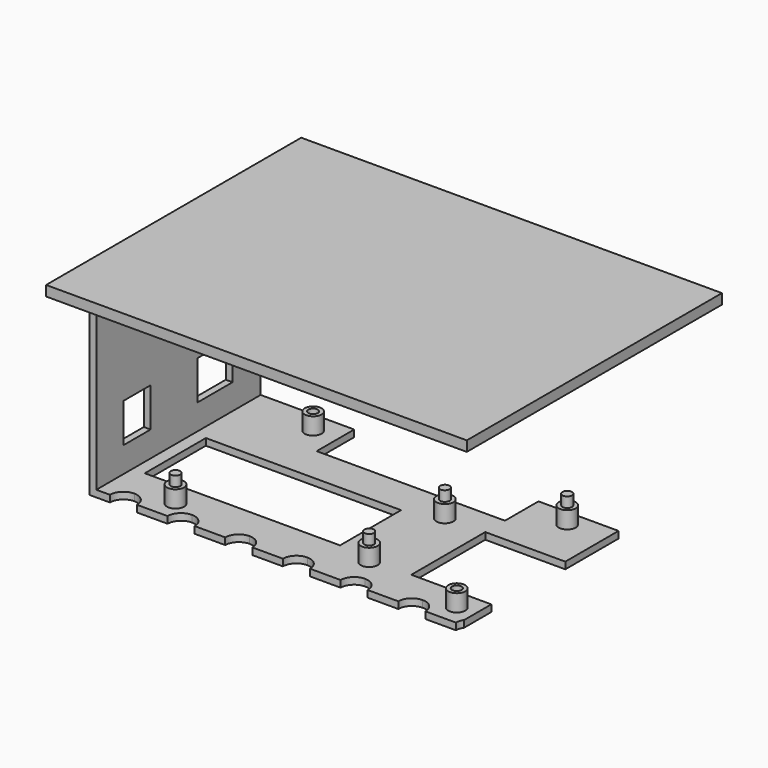
from build123d import *

# Parameters (mm, degrees)
F0_W      = 124
F0_H      = 94
F1_DEPTH  = 2
F2_DEPTH  = 58
F3_R      = 2.5
F4_DEPTH  = 5
F5_R      = 1.4
F6_DEPTH  = 3
F7_D      = 2.8
F7_DEPTH  = 5
F7_TIP    = 0.8412048666
F9_DEPTH  = 8
F10_W     = 1
F10_H     = 50
F11_DEPTH = 3
F12_W     = 5
F12_H     = 3
F13_DEPTH = 1
F14_W     = 124
F14_H     = 94
F15_DEPTH = 3
F17_W     = 2
F17_H     = 13
F17_H_2   = 10
F18_DEPTH = 11.5
F19_W     = 199.5194256306
F19_H     = 143.535412848
F19_W_2   = 57.5444861315
F19_H_2   = 22.4794349963
F20_DEPTH = 100


# Not quite as in the source:
# - a feature names something its author has since deleted; it is built from what else it names


with BuildPart() as f1:
    # F0 (on Top) → F1 (new body)
    with BuildSketch(Plane.XY):
        Rectangle(F0_W, F0_H)
        Polygon((-60, -45), (-60, 45), (60, 45), (60, 31), (60, 29), (60, -45), align=None, mode=Mode.SUBTRACT)
        Polygon((60, 45), (-60, 45), (-60, -45), (60, -45), (60, 29), (60, 31), align=None)
    extrude(amount=F1_DEPTH)

    # F0 (on Top) → F2 (join)
    with BuildSketch(Plane.XY):
        Rectangle(F0_W, F0_H)
        Polygon((-60, -45), (-60, 45), (60, 45), (60, 31), (60, 29), (60, -45), align=None, mode=Mode.SUBTRACT)
    extrude(amount=F2_DEPTH)

    # F3 (on face) → F4 (join)
    with BuildSketch(Plane.XY.offset(2)):
        with Locations((35.45, 23.2)):
            Circle(F3_R)
        with Locations((11.55, -19.9)):
            Circle(F3_R)
        with Locations((41.45, -25)):
            Circle(F3_R)
        with Locations((11.55, 8)):
            Circle(F3_R)
        with Locations((-39.45, 23.2)):
            Circle(F3_R)
        with Locations((-41.45, -25)):
            Circle(F3_R)
    extrude(amount=F4_DEPTH)

    # F5 (on face) → F6 (join)
    with BuildSketch(Plane.XY.offset(7)):
        with Locations((35.45, 23.2)):
            Circle(F5_R)
        with Locations((11.55, 8)):
            Circle(F5_R)
        with Locations((11.55, -19.9)):
            Circle(F5_R)
        with Locations((-41.45, -25)):
            Circle(F5_R)
    extrude(amount=F6_DEPTH)

    # F7 (one way)
    with BuildSketch(Plane(origin=(0, 0, 2), x_dir=(1, 0, 0), z_dir=(0, 0, -1))):
        with Locations((-39.45, -23.2), (41.45, 25)):
            Circle(F7_D / 2)
    extrude(amount=-F7_DEPTH, mode=Mode.SUBTRACT)
    with Locations(Plane(origin=(0, 0, 2), x_dir=(1, 0, 0), z_dir=(0, 0, -1))):
        with Locations((-39.45, -23.2), (41.45, 25)):
            with Locations((0, 0, -(F7_DEPTH + F7_TIP / 2))):  # 118° drill point
                Cone(0, F7_D / 2, F7_TIP, mode=Mode.SUBTRACT)

    # F8 (on face) → F9 (cut)
    with BuildSketch(Plane(origin=(0, 0, 0), x_dir=(1, 0, 0), z_dir=(0, 0, -1))):
        with BuildLine():
            Line((-52, 27), (-52, 47))
            Line((-52, 47), (-56, 47))
            Line((-56, 47), (-56, 31))
            ThreePointArc((-56, 31), (-54.8284271247, 28.1715728753), (-52, 27))
        make_face()
        with BuildLine():
            Line((-48, 47), (-52, 47))
            Line((-52, 47), (-52, 27))
            ThreePointArc((-52, 27), (-49.1715728753, 28.1715728753), (-48, 31))
            Line((-48, 31), (-48, 47))
        make_face()
        with BuildLine():
            Line((-35, 47), (-39, 47))
            Line((-39, 47), (-39, 31))
            ThreePointArc((-39, 31), (-37.8284271247, 28.1715728753), (-35, 27))
            ThreePointArc((-35, 27), (-32.1715728753, 28.1715728753), (-31, 31))
            Line((-31, 31), (-31, 47))
            Line((-31, 47), (-35, 47))
        make_face()
        with BuildLine():
            Line((-18, 47), (-22, 47))
            Line((-22, 47), (-22, 31))
            ThreePointArc((-22, 31), (-20.8284271247, 28.1715728753), (-18, 27))
            ThreePointArc((-18, 27), (-15.1715728753, 28.1715728753), (-14, 31))
            Line((-14, 31), (-14, 47))
            Line((-14, 47), (-18, 47))
        make_face()
        with BuildLine():
            Line((-1, 47), (-5, 47))
            Line((-5, 47), (-5, 31))
            ThreePointArc((-5, 31), (-3.8284271247, 28.1715728753), (-1, 27))
            ThreePointArc((-1, 27), (1.8284271247, 28.1715728753), (3, 31))
            Line((3, 31), (3, 47))
            Line((3, 47), (-1, 47))
        make_face()
        with BuildLine():
            Line((16, 47), (12, 47))
            Line((12, 47), (12, 31))
            ThreePointArc((12, 31), (13.1715728753, 28.1715728753), (16, 27))
            ThreePointArc((16, 27), (18.8284271247, 28.1715728753), (20, 31))
            Line((20, 31), (20, 47))
            Line((20, 47), (16, 47))
        make_face()
        with BuildLine():
            Line((37, 31), (37, 47))
            Line((37, 47), (33, 47))
            Line((33, 47), (29, 47))
            Line((29, 47), (29, 31))
            ThreePointArc((29, 31), (30.1715728753, 28.1715728753), (33, 27))
            ThreePointArc((33, 27), (35.8284271247, 28.1715728753), (37, 31))
        make_face()
        with BuildLine():
            Line((54, 31), (54, 47))
            Line((54, 47), (50, 47))
            Line((50, 47), (46, 47))
            Line((46, 47), (46, 31))
            ThreePointArc((46, 31), (47.1715728753, 28.1715728753), (50, 27))
            ThreePointArc((50, 27), (52.8284271247, 28.1715728753), (54, 31))
        make_face()
    extrude(amount=-F9_DEPTH, mode=Mode.SUBTRACT)

    # F10 (on face) → F11 (join)
    with BuildSketch(Plane.XZ.offset(-45)):
        with Locations((-42, 27)):
            Rectangle(F10_W, F10_H)
        with Locations((-38, 27)):
            Rectangle(F10_W, F10_H)
        with Locations((2, 27)):
            Rectangle(F10_W, F10_H)
        with Locations((-2, 27)):
            Rectangle(F10_W, F10_H)
        with Locations((38, 27)):
            Rectangle(F10_W, F10_H)
        with Locations((42, 27)):
            Rectangle(F10_W, F10_H)
    extrude(amount=F11_DEPTH)

    # F12 (on face) → F13 (join)
    with BuildSketch(Plane.XZ.offset(-42)):
        with Locations((0, 50.5)):
            Rectangle(F12_W, F12_H)
        with Locations((0, 42.5)):
            Rectangle(F12_W, F12_H)
        with Locations((0, 35.5)):
            Rectangle(F12_W, F12_H)
        with Locations((0, 27.5)):
            Rectangle(F12_W, F12_H)
        with Locations((0, 19.5)):
            Rectangle(F12_W, F12_H)
        with Locations((0, 11.5)):
            Rectangle(F12_W, F12_H)
        with Locations((40, 19.5)):
            Rectangle(F12_W, F12_H)
        with Locations((40, 42.5)):
            Rectangle(F12_W, F12_H)
        with Locations((40, 50.5)):
            Rectangle(F12_W, F12_H)
        with Locations((40, 35.5)):
            Rectangle(F12_W, F12_H)
        with Locations((40, 27.5)):
            Rectangle(F12_W, F12_H)
        with Locations((40, 11.5)):
            Rectangle(F12_W, F12_H)
        with Locations((-40, 19.5)):
            Rectangle(F12_W, F12_H)
        with Locations((-40, 50.5)):
            Rectangle(F12_W, F12_H)
        with Locations((-40, 27.5)):
            Rectangle(F12_W, F12_H)
        with Locations((-40, 35.5)):
            Rectangle(F12_W, F12_H)
        with Locations((-40, 11.5)):
            Rectangle(F12_W, F12_H)
        with Locations((-40, 42.5)):
            Rectangle(F12_W, F12_H)
    extrude(amount=-F13_DEPTH)

    # F17 (on offset) → F18 (cut)
    with BuildSketch(Plane.XY.offset(9.5)):
        with Locations((-61, 12.7)):
            Rectangle(F17_W, F17_H)
        with Locations((-61, -16)):
            Rectangle(F17_W, F17_H_2)
    extrude(amount=F18_DEPTH, mode=Mode.SUBTRACT)

    # F19 (on Top) → F20 (cut)
    with BuildSketch(Plane.XY):
        with Locations((2.5972127914, -1.2879259884)):
            Rectangle(F19_W, F19_H)
        Polygon((-68.1005078713, -30.994397391), (-68.1005078713, 29.5461390275), (-32.4154566388, 29.5461390275), (-32.4154566388, 15.7205138463), (23.0738711198, 15.7205138463), (23.0738711198, 28.0771622352), (46.6675695452, 28.0771622352), (46.6675695452, 8.4633265807), (23.0738711198, 8.4633265807), (23.0738711198, -18.7967714509), (46.6675695452, -18.7967714509), (46.6675695452, -30.994397391), align=None, mode=Mode.SUBTRACT)
        with Locations((-27.6512478013, -6.3523130957)):
            Rectangle(F19_W_2, F19_H_2)
    extrude(amount=F20_DEPTH, mode=Mode.SUBTRACT)


with BuildPart() as f15:
    # F14 (on face) → F15 (new body)
    with BuildSketch(Plane.XY.offset(58)):
        Rectangle(F14_W, F14_H)
    extrude(amount=F15_DEPTH)


solid = Compound([f1.part, f15.part])
